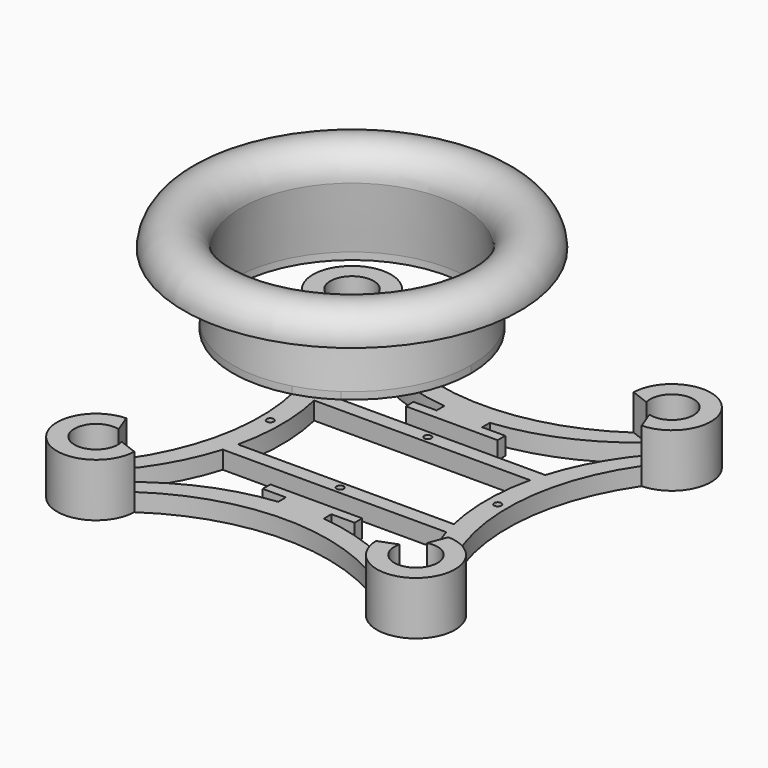
from build123d import *

# Parameters (mm, degrees)
F1_DEPTH = 2.5
F3_DEPTH = 5
F4_R     = 0.5
F5_DEPTH = 25
F7_DEPTH = 2.5
F9_DEPTH = 1


# Not quite as in the source:
# - a feature names something its author has since deleted; it is built from what else it names


with BuildPart() as f1:
    # F0 (on Top) → F1 (new body)
    with BuildSketch(Plane.XY):
        with BuildLine():
            ThreePointArc((-17.0023033122, 22.6591575617), (-26.3890872965, 26.3890872965), (-22.6591575617, 17.0023033122))
            ThreePointArc((-22.6591575617, 17.0023033122), (-17.3759874976, 0), (-22.6591575617, -17.0023033122))
            ThreePointArc((-22.6591575617, -17.0023033122), (-26.3890872965, -26.3890872965), (-17.0023033122, -22.6591575617))
            ThreePointArc((-17.0023033122, -22.6591575617), (0, -17.3759874976), (17.0023033122, -22.6591575617))
            ThreePointArc((17.0023033122, -22.6591575617), (26.3890872965, -26.3890872965), (22.6591575617, -17.0023033122))
            ThreePointArc((22.6591575617, -17.0023033122), (17.3759874976, 0), (22.6591575617, 17.0023033122))
            ThreePointArc((22.6591575617, 17.0023033122), (26.3890872965, 26.3890872965), (17.0023033122, 22.6591575617))
            ThreePointArc((17.0023033122, 22.6591575617), (0, 17.3759874976), (-17.0023033122, 22.6591575617))
        make_face()
        with BuildLine():
            ThreePointArc((-21.682828976, 19.5615086324), (-24.9284636731, 24.3452816014), (-19.45, 22.5))
            ThreePointArc((-19.45, 22.5), (-19.4780057353, 22.0876280024), (-19.5615086324, 21.682828976))
            ThreePointArc((-19.5615086324, 21.682828976), (0, 14.428100573), (19.5615086324, 21.682828976))
            ThreePointArc((19.5615086324, 21.682828976), (22.0876280024, 25.5219942647), (25.55, 22.5))
            ThreePointArc((25.55, 22.5), (24.3452816014, 20.0715363269), (21.682828976, 19.5615086324))
            ThreePointArc((21.682828976, 19.5615086324), (18.1332032787, 14.4422427718), (15.7173763175, 8.700247854))
            ThreePointArc((15.7173763175, 8.700247854), (15.4343846251, 7.7048319598), (15.1858934283, 6.700247854))
            ThreePointArc((15.1858934283, 6.700247854), (14.428100573, 0), (15.1858934283, -6.700247854))
            ThreePointArc((15.1858934283, -6.700247854), (15.4343846251, -7.7048319598), (15.7173763175, -8.700247854))
            ThreePointArc((15.7173763175, -8.700247854), (18.1332032787, -14.4422427718), (21.682828976, -19.5615086324))
            ThreePointArc((21.682828976, -19.5615086324), (24.3452816014, -20.0715363269), (25.55, -22.5))
            ThreePointArc((25.55, -22.5), (22.0876280024, -25.5219942647), (19.5615086324, -21.682828976))
            ThreePointArc((19.5615086324, -21.682828976), (0, -14.428100573), (-19.5615086324, -21.682828976))
            ThreePointArc((-19.5615086324, -21.682828976), (-19.4780057353, -22.0876280024), (-19.45, -22.5))
            ThreePointArc((-19.45, -22.5), (-24.9284636731, -24.3452816014), (-21.682828976, -19.5615086324))
            ThreePointArc((-21.682828976, -19.5615086324), (-18.1332032787, -14.4422427718), (-15.7173763175, -8.700247854))
            ThreePointArc((-15.7173763175, -8.700247854), (-15.4343846251, -7.7048319598), (-15.1858934283, -6.700247854))
            ThreePointArc((-15.1858934283, -6.700247854), (-14.428100573, 0), (-15.1858934283, 6.700247854))
            ThreePointArc((-15.1858934283, 6.700247854), (-15.4343846251, 7.7048319598), (-15.7173763175, 8.700247854))
            ThreePointArc((-15.7173763175, 8.700247854), (-18.1332032787, 14.4422427718), (-21.682828976, 19.5615086324))
        make_face(mode=Mode.SUBTRACT)
        with BuildLine():
            Line((15.7173763175, 8.700247854), (-15.7173763175, 8.700247854))
            ThreePointArc((-15.7173763175, 8.700247854), (-15.4343846251, 7.7048319598), (-15.1858934283, 6.700247854))
            Line((-15.1858934283, 6.700247854), (15.1858934283, 6.700247854))
            ThreePointArc((15.1858934283, 6.700247854), (15.4343846251, 7.7048319598), (15.7173763175, 8.700247854))
        make_face()
        with BuildLine():
            Line((15.1858934283, -6.700247854), (-15.1858934283, -6.700247854))
            ThreePointArc((-15.1858934283, -6.700247854), (-15.4343846251, -7.7048319598), (-15.7173763175, -8.700247854))
            Line((-15.7173763175, -8.700247854), (15.7173763175, -8.700247854))
            ThreePointArc((15.7173763175, -8.700247854), (15.4343846251, -7.7048319598), (15.1858934283, -6.700247854))
        make_face()
    extrude(amount=F1_DEPTH)

    # F2 (on face) → F3 (join)
    with BuildSketch(Plane.XY.offset(2.5)):
        with BuildLine():
            ThreePointArc((-21.682828976, 19.5615086324), (-24.6566756826, 24.6566756826), (-19.5615086324, 21.682828976))
            Line((-19.5615086324, 21.682828976), (-17.0023033122, 22.6591575617))
            ThreePointArc((-17.0023033122, 22.6591575617), (-26.3890872965, 26.3890872965), (-22.6591575617, 17.0023033122))
            Line((-22.6591575617, 17.0023033122), (-21.682828976, 19.5615086324))
        make_face()
        with BuildLine():
            Line((-21.682828976, -19.5615086324), (-22.6591575617, -17.0023033122))
            ThreePointArc((-22.6591575617, -17.0023033122), (-26.3890872965, -26.3890872965), (-17.0023033122, -22.6591575617))
            Line((-17.0023033122, -22.6591575617), (-19.5615086324, -21.682828976))
            ThreePointArc((-19.5615086324, -21.682828976), (-24.6566756826, -24.6566756826), (-21.682828976, -19.5615086324))
        make_face()
        with BuildLine():
            ThreePointArc((17.0023033122, -22.6591575617), (26.3890872965, -26.3890872965), (22.6591575617, -17.0023033122))
            Line((22.6591575617, -17.0023033122), (21.682828976, -19.5615086324))
            ThreePointArc((21.682828976, -19.5615086324), (24.6566756826, -24.6566756826), (19.5615086324, -21.682828976))
            Line((19.5615086324, -21.682828976), (17.0023033122, -22.6591575617))
        make_face()
        with BuildLine():
            Line((17.0023033122, 22.6591575617), (19.5615086324, 21.682828976))
            ThreePointArc((19.5615086324, 21.682828976), (24.6566756826, 24.6566756826), (21.682828976, 19.5615086324))
            Line((21.682828976, 19.5615086324), (22.6591575617, 17.0023033122))
            ThreePointArc((22.6591575617, 17.0023033122), (26.3890872965, 26.3890872965), (17.0023033122, 22.6591575617))
        make_face()
    extrude(amount=F3_DEPTH)

    # F4 (on face) → F5 (cut)
    with BuildSketch(Plane.XY.offset(2.5)):
        with Locations((16, 0)):
            Circle(F4_R)
        with Locations((-16, 0)):
            Circle(F4_R)
        with Locations((0, 7.700247854)):
            Circle(F4_R)
        with Locations((0, -7.700247854)):
            Circle(F4_R)
    extrude(amount=-F5_DEPTH, mode=Mode.SUBTRACT)

    # F6 (on face) → F7 (join, through all)
    with BuildSketch(Plane(origin=(0, 0, 0), x_dir=(1, 0, 0), z_dir=(0, 0, -1))):
        with BuildLine():
            Line((-3.2028362621, -13.2521484047), (-3.2028362621, -14.59955988))
            ThreePointArc((-3.2028362621, -14.59955988), (0, -14.428100573), (3.2028362621, -14.59955988))
            Line((3.2028362621, -14.59955988), (3.2028362621, -13.2521484047))
            Line((3.2028362621, -13.2521484047), (6.4590500986, -13.2521484047))
            Line((6.4590500986, -13.2521484047), (6.4590500986, -11.9047369295))
            Line((6.4590500986, -11.9047369295), (-6.4590500986, -11.9047369295))
            Line((-6.4590500986, -11.9047369295), (-6.4590500986, -13.2521484047))
            Line((-6.4590500986, -13.2521484047), (-3.2028362621, -13.2521484047))
        make_face()
        with BuildLine():
            Line((3.2028362621, 13.2521484047), (3.2028362621, 14.59955988))
            ThreePointArc((3.2028362621, 14.59955988), (0, 14.428100573), (-3.2028362621, 14.59955988))
            Line((-3.2028362621, 14.59955988), (-3.2028362621, 13.2521484047))
            Line((-3.2028362621, 13.2521484047), (-6.4590500986, 13.2521484047))
            Line((-6.4590500986, 13.2521484047), (-6.4590500986, 11.9047369295))
            Line((-6.4590500986, 11.9047369295), (6.4590500986, 11.9047369295))
            Line((6.4590500986, 11.9047369295), (6.4590500986, 13.2521484047))
            Line((6.4590500986, 13.2521484047), (3.2028362621, 13.2521484047))
        make_face()
    extrude(amount=-F7_DEPTH)


with BuildPart() as f9:
    # F8 (on face) → F9 (new body)
    with BuildSketch(Plane.XY.offset(2.5)):
        with BuildLine():
            ThreePointArc((-18.1098129291, 6.5947726366), (-20.5216852868, 6.1190271688), (-22.9774726852, 6.0069099367))
            ThreePointArc((-22.9774726852, 6.0069099367), (-23.6964367213, 6.0434347699), (-24.4131232722, 6.1112856104))
            ThreePointArc((-24.4131232722, 6.1112856104), (-34.1672618896, 34.1672618896), (-6.1112856104, 24.4131232722))
            ThreePointArc((-6.1112856104, 24.4131232722), (-6.0434347699, 23.6964367213), (-6.0069099367, 22.9774726852))
            ThreePointArc((-6.0069099367, 22.9774726852), (-6.0017275746, 22.7387613413), (-6, 22.5))
            ThreePointArc((-6, 22.5), (-7.9828223753, 14.6577073624), (-13.4547337956, 8.700247854))
            Line((-13.4547337956, 8.700247854), (-13.006352613, 8.700247854))
            ThreePointArc((-13.006352613, 8.700247854), (-7.6746653709, 14.704363199), (-5.75, 22.5))
            ThreePointArc((-5.75, 22.5), (-35.8229651319, 32.6519013044), (-18.0558029963, 6.3503370626))
            ThreePointArc((-18.0558029963, 6.3503370626), (-18.0825530037, 6.4726111847), (-18.1098129291, 6.5947726366))
        make_face()
        with BuildLine():
            ThreePointArc((-13.4547337956, 8.700247854), (-15.7002862082, 7.4662415761), (-18.1098129291, 6.5947726366))
            ThreePointArc((-18.1098129291, 6.5947726366), (-18.0825530037, 6.4726111847), (-18.0558029963, 6.3503370626))
            ThreePointArc((-18.0558029963, 6.3503370626), (-15.4327235269, 7.3139503737), (-13.006352613, 8.700247854))
            Line((-13.006352613, 8.700247854), (-13.4547337956, 8.700247854))
        make_face()
        with BuildLine():
            Line((-6.1112856104, 24.4131232722), (-16.0438397859, 23.2536546224))
            ThreePointArc((-16.0438397859, 23.2536546224), (-16.0171106669, 22.9713235569), (-16.0027220963, 22.6880953002))
            Line((-16.0027220963, 22.6880953002), (-6.0069099367, 22.9774726852))
            ThreePointArc((-6.0069099367, 22.9774726852), (-6.0434347699, 23.6964367213), (-6.1112856104, 24.4131232722))
        make_face()
        with BuildLine():
            Line((-22.9774726852, 6.0069099367), (-22.6880953002, 16.0027220963))
            ThreePointArc((-22.6880953002, 16.0027220963), (-22.9713235569, 16.0171106669), (-23.2536546224, 16.0438397859))
            Line((-23.2536546224, 16.0438397859), (-24.4131232722, 6.1112856104))
            ThreePointArc((-24.4131232722, 6.1112856104), (-23.6964367213, 6.0434347699), (-22.9774726852, 6.0069099367))
        make_face()
        with BuildLine():
            Line((-23.2536546224, 16.0438397859), (-23.1377077574, 17.0370952035))
            ThreePointArc((-23.1377077574, 17.0370952035), (-26.3890872965, 26.3890872965), (-17.0370952035, 23.1377077574))
            Line((-17.0370952035, 23.1377077574), (-16.0438397859, 23.2536546224))
            ThreePointArc((-16.0438397859, 23.2536546224), (-27.0961940777, 27.0961940777), (-23.2536546224, 16.0438397859))
        make_face()
        with BuildLine():
            Line((-22.6880953002, 16.0027220963), (-22.6591575617, 17.0023033122))
            ThreePointArc((-22.6591575617, 17.0023033122), (-22.8988122404, 17.0144782566), (-23.1377077574, 17.0370952035))
            Line((-23.1377077574, 17.0370952035), (-23.2536546224, 16.0438397859))
            ThreePointArc((-23.2536546224, 16.0438397859), (-22.9713235569, 16.0171106669), (-22.6880953002, 16.0027220963))
        make_face()
        with BuildLine():
            Line((-16.0438397859, 23.2536546224), (-17.0370952035, 23.1377077574))
            ThreePointArc((-17.0370952035, 23.1377077574), (-17.0144782566, 22.8988122404), (-17.0023033122, 22.6591575617))
            Line((-17.0023033122, 22.6591575617), (-16.0027220963, 22.6880953002))
            ThreePointArc((-16.0027220963, 22.6880953002), (-16.0171106669, 22.9713235569), (-16.0438397859, 23.2536546224))
        make_face()
        with BuildLine():
            ThreePointArc((-22.0198246983, 16.0332469604), (-22.3348030624, 16.520868079), (-22.6591575617, 17.0023033122))
            Line((-22.6591575617, 17.0023033122), (-22.6880953002, 16.0027220963))
            Line((-22.6880953002, 16.0027220963), (-22.9774726852, 6.0069099367))
            Line((-22.9774726852, 6.0069099367), (-22.0198246983, 16.0332469604))
        make_face()
        with BuildLine():
            Line((-21.682828976, 19.5615086324), (-22.6591575617, 17.0023033122))
            ThreePointArc((-22.6591575617, 17.0023033122), (-22.3348030624, 16.520868079), (-22.0198246983, 16.0332469604))
            Line((-22.0198246983, 16.0332469604), (-21.682828976, 19.5615086324))
        make_face()
        Polygon((-16.0027220963, 22.6880953002), (-17.0023033122, 22.6591575617), (-19.5615086324, 21.682828976), (-6.0069099367, 22.9774726852), align=None)
    extrude(amount=F9_DEPTH)

    # F12 (on line) → F13 (revolve)
    with BuildSketch(Plane.YZ.offset(-22.5)):
        with BuildLine():
            Line((38.1, 12.5), (39, 3.5))
            Line((39, 3.5), (39.25, 3.5))
            Line((39.25, 3.5), (38.35, 12.5))
            ThreePointArc((38.35, 12.5), (42.25344, 16.3154189444), (46.15688, 12.5))
            ThreePointArc((46.15688, 12.5), (42.12844, 16.52844), (38.1, 12.5))
        make_face()
    revolve(axis=Axis((-22.5, 22.5, 14.4747497439), (0, 0, 1)))


solid = Compound([f1.part, f9.part])
